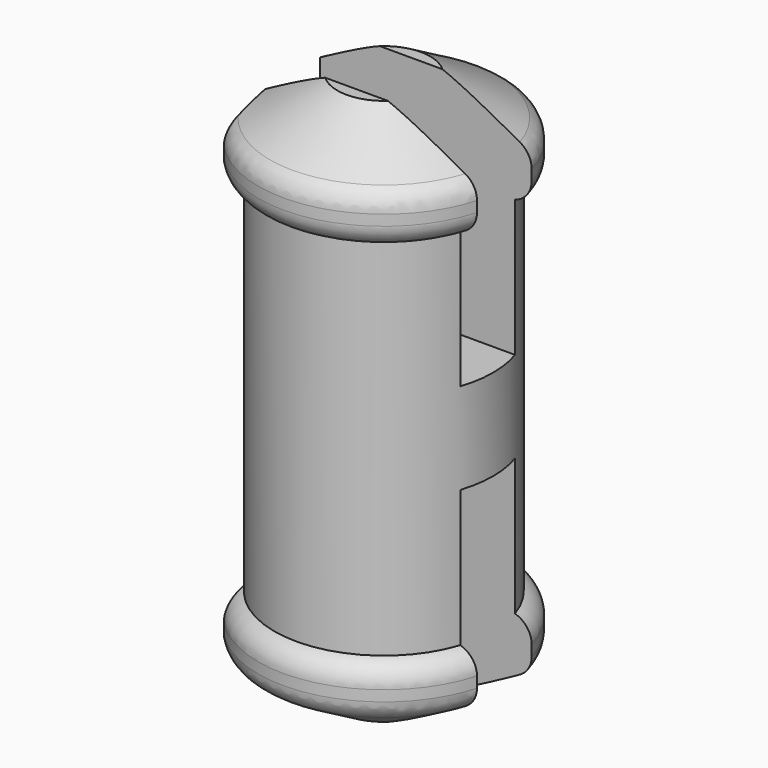
from build123d import *

# Parameters (mm, degrees)
F0_R         = 2.75
F1_DEPTH     = 2
F2_R         = 2.4
F3_DEPTH     = 8
F4_R         = 2.75
F5_DEPTH     = 2
F8_DEPTH     = 5
F10_DEPTH    = 5
F11_C1_SIZE2 = 1
F11_C1_SIZE  = 1.7320508076
F11_C2_SIZE2 = 1
F11_C2_SIZE  = 1.7320508076
F12_C1_SIZE2 = 1
F12_C1_SIZE  = 1.7320508076
F12_C2_SIZE2 = 1
F12_C2_SIZE  = 1.7320508076
F13_R        = 0.5
F15_DEPTH    = 25


# Not quite as in the source:
# - a fillet or chamfer that OpenCascade refuses, or shapes differently, is made with other operations: its cross-section is extruded or revolved along the edge and cut away or added


with BuildPart() as f1:
    # F0 (on Top) → F1 (new body)
    with BuildSketch(Plane.XY):
        Circle(F0_R)
    extrude(amount=F1_DEPTH)

    # F2 (on face) → F3 (join)
    with BuildSketch(Plane.XY.offset(2)):
        Circle(F2_R)
    extrude(amount=F3_DEPTH)

    # F4 (on face) → F5 (join)
    with BuildSketch(Plane.XY.offset(10)):
        Circle(F4_R)
    extrude(amount=F5_DEPTH)

    # F6: fillet of radius 0.5 on 2 edges, made by hand

    # F6_s1 → F6_t2 (revolve, cut)
    with BuildSketch(Plane.XZ):
        with BuildLine():
            ThreePointArc((2.4, 2), (2.6531128874, 1.8188343884), (2.75, 1.5230303993))
            Line((2.75, 1.5230303993), (2.75, 2))
            Line((2.75, 2), (2.4, 2))
        make_face()
    revolve(axis=Axis((0, 0, 2), (0, 0, 1)), mode=Mode.SUBTRACT)

    # F6_s3 → F6_t4 (revolve, cut)
    with BuildSketch(Plane.XZ):
        with BuildLine():
            ThreePointArc((2.75, 10.4769696007), (2.6531128874, 10.1811656116), (2.4, 10))
            Line((2.4, 10), (2.75, 10))
            Line((2.75, 10), (2.75, 10.4769696007))
        make_face()
    revolve(axis=Axis((0, 0, 10), (0, 0, 1)), mode=Mode.SUBTRACT)

    # F7 (on face) → F8 (cut)
    with BuildSketch(Plane(origin=(0, 0, 0), x_dir=(1, 0, 0), z_dir=(0, 0, -1))):
        with BuildLine():
            ThreePointArc((-2.6457513111, 0.75), (-2.75, 0), (-2.6457513111, -0.75))
            Line((-2.6457513111, -0.75), (2.6457513111, -0.75))
            ThreePointArc((2.6457513111, -0.75), (2.75, 0), (2.6457513111, 0.75))
            Line((2.6457513111, 0.75), (-2.6457513111, 0.75))
        make_face()
    extrude(amount=-F8_DEPTH, mode=Mode.SUBTRACT)

    # F9 (on face) → F10 (cut)
    with BuildSketch(Plane.XY.offset(12)):
        with BuildLine():
            ThreePointArc((-2.6457513111, 0.75), (-2.75, 0), (-2.6457513111, -0.75))
            Line((-2.6457513111, -0.75), (2.6457513111, -0.75))
            ThreePointArc((2.6457513111, -0.75), (2.75, 0), (2.6457513111, 0.75))
            Line((2.6457513111, 0.75), (-2.6457513111, 0.75))
        make_face()
    extrude(amount=-F10_DEPTH, mode=Mode.SUBTRACT)

    # F11: chamfer of 1 x 1.7320508076 on 2 edges, made by hand

    # F11_c1
    f11_c1_edges = [f1.edges().sort_by_distance(p)[0] for p in [
        (0, 2.75, 0),
    ]]
    f11_c1_side = f1.faces().sort_by_distance((0, 2.73, 0))[0]
    chamfer(f11_c1_edges, length=F11_C1_SIZE, length2=F11_C1_SIZE2, reference=f11_c1_side)

    # F11_c2
    f11_c2_edges = [f1.edges().sort_by_distance(p)[0] for p in [
        (0, -2.75, 0),
    ]]
    f11_c2_side = f1.faces().sort_by_distance((0, -2.73, 0))[0]
    chamfer(f11_c2_edges, length=F11_C2_SIZE, length2=F11_C2_SIZE2, reference=f11_c2_side)

    # F12: chamfer of 1 x 1.7320508076 on 2 edges, made by hand

    # F12_c1
    f12_c1_edges = [f1.edges().sort_by_distance(p)[0] for p in [
        (0, -2.75, 12),
    ]]
    f12_c1_side = f1.faces().sort_by_distance((0, -2.73, 12))[0]
    chamfer(f12_c1_edges, length=F12_C1_SIZE, length2=F12_C1_SIZE2, reference=f12_c1_side)

    # F12_c2
    f12_c2_edges = [f1.edges().sort_by_distance(p)[0] for p in [
        (0, 2.75, 12),
    ]]
    f12_c2_side = f1.faces().sort_by_distance((0, 2.73, 12))[0]
    chamfer(f12_c2_edges, length=F12_C2_SIZE, length2=F12_C2_SIZE2, reference=f12_c2_side)

    # F13
    f13_edges = [f1.edges().sort_by_distance(p)[0] for p in [
        (0, -2.75, 11),
        (0, 2.75, 11),
        (0, -2.75, 1),
        (0, 2.75, 1),
    ]]
    fillet(f13_edges, radius=F13_R)

    # F14 (on face) → F15 (cut)
    with BuildSketch(Plane.XY.offset(12)):
        with BuildLine():
            Line((-2, -1.8874586088), (-2, 1.8874586088))
            ThreePointArc((-2, 1.8874586088), (-2.75, 0), (-2, -1.8874586088))
        make_face()
    extrude(amount=-F15_DEPTH, mode=Mode.SUBTRACT)


solid = f1.part
